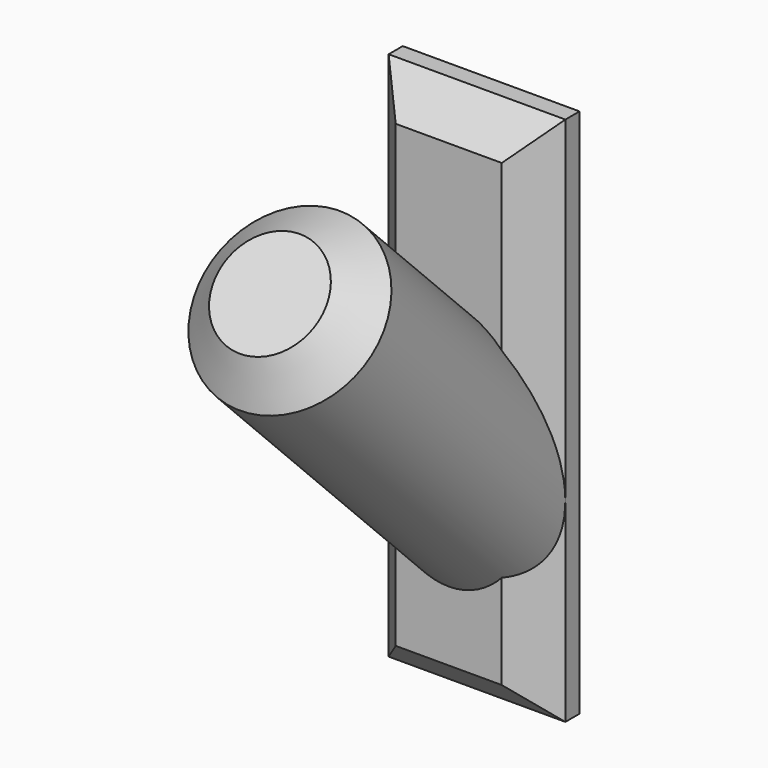
from build123d import *

# Parameters (mm, degrees)
F0_W          = 10
F0_H          = 30
F1_DEPTH      = 3
F4_R          = 5
F5_DEPTH      = 20
F5_DEPTH_BACK = 5
F6_T1_DEPTH   = 20.2867319519
F6_T6_DEPTH   = 22.1433659759
F6_S7_R       = 5
F6_T8_DEPTH   = 13
F6_T14_DEPTH  = 22.1433659759
F6_S15_R      = 5
F6_T16_DEPTH  = 13
F6_T20_DEPTH  = 18.1433659759
F6_S21_R      = 5
F6_T22_DEPTH  = 11
F6_T26_DEPTH  = 18.1433659759
F6_S27_R      = 5
F6_T28_DEPTH  = 11
F7_DEPTH      = 25


# Not quite as in the source:
# - a fillet or chamfer that OpenCascade refuses, or shapes differently, is made with other operations: its cross-section is extruded or revolved along the edge and cut away or added


with BuildPart() as f1:
    # F0 (on Front) → F1 (new body)
    with BuildSketch(Plane.XZ):
        with Locations((0, 5)):
            Rectangle(F0_W, F0_H)
    extrude(amount=F1_DEPTH)

    # F4 (on face) → F5 (join, two sides)
    with BuildSketch(Plane(origin=(0, -1.5, 1.5), x_dir=(1, 0, 0), z_dir=(0, -0.7071067812, 0.7071067812))) as f5_sk:
        Circle(F4_R)
    extrude(amount=F5_DEPTH)
    extrude(f5_sk.sketch, amount=-F5_DEPTH_BACK)

    # F6: chamfer of 2 on 5 edges, made by hand

    # F6_s2 → F6_t1 (cut)
    with BuildSketch(Plane.YZ.offset(-10.1433659759)):
        Polygon((-1, 20), (-3, 18), (-3, 20), align=None)
        Polygon((-3, -8), (-1, -10), (-3, -10), align=None)
    extrude(amount=F6_T1_DEPTH, mode=Mode.SUBTRACT)


with BuildPart() as f6_tool4:
    # F6_s5 → F6_t6 (new body)
    with BuildSketch(Plane.XY.offset(25.1433659759)):
        Polygon((-3, -3), (-5, -1), (-5, -3), align=None)
    extrude(amount=-F6_T6_DEPTH)

    # F6_s7 → F6_t8 (cut, symmetric)
    with BuildSketch(Plane(origin=(0, -8.0610173055, 8.0610173055), x_dir=(1, 0, 0), z_dir=(0, 0.7071067812, -0.7071067812))):
        Circle(F6_S7_R)
    extrude(amount=F6_T8_DEPTH, both=True, mode=Mode.SUBTRACT)


with BuildPart() as f1_1:
    add(f1.part)

    # F6_t3: cut F6_tool4
    add(f6_tool4.part, mode=Mode.SUBTRACT)

    # F6_s9 → F6_t10 (revolve, cut)
    with BuildSketch(Plane(origin=(0, 0, 0), x_dir=(1, 0, 0), z_dir=(0, -0.7071067812, -0.7071067812))):
        Polygon((5, 20.1213203436), (3, 22.1213203436), (5, 22.1213203436), align=None)
    revolve(axis=Axis((0, -15.6421356237, 15.6421356237), (0, -0.7071067812, 0.7071067812)), mode=Mode.SUBTRACT)


with BuildPart() as f6_tool12:
    # F6_s13 → F6_t14 (new body)
    with BuildSketch(Plane.XY.offset(3)):
        Polygon((3, -3), (5, -1), (5, -3), align=None)
    extrude(amount=F6_T14_DEPTH)

    # F6_s15 → F6_t16 (cut, symmetric)
    with BuildSketch(Plane(origin=(0, -8.0610173055, 8.0610173055), x_dir=(1, 0, 0), z_dir=(0, 0.7071067812, -0.7071067812))):
        Circle(F6_S15_R)
    extrude(amount=F6_T16_DEPTH, both=True, mode=Mode.SUBTRACT)


with BuildPart() as f1_2:
    add(f1_1.part)

    # F6_t11: cut F6_tool12
    add(f6_tool12.part, mode=Mode.SUBTRACT)


with BuildPart() as f6_tool18:
    # F6_s19 → F6_t20 (new body)
    with BuildSketch(Plane.XY.offset(-15.1433659759)):
        Polygon((3, -3), (5, -1), (5, -3), align=None)
    extrude(amount=F6_T20_DEPTH)

    # F6_s21 → F6_t22 (cut, symmetric)
    with BuildSketch(Plane(origin=(0, 2.0506096654, -2.0506096654), x_dir=(1, 0, 0), z_dir=(0, 0.7071067812, -0.7071067812))):
        Circle(F6_S21_R)
    extrude(amount=F6_T22_DEPTH, both=True, mode=Mode.SUBTRACT)


with BuildPart() as f1_3:
    add(f1_2.part)

    # F6_t17: cut F6_tool18
    add(f6_tool18.part, mode=Mode.SUBTRACT)


with BuildPart() as f6_tool24:
    # F6_s25 → F6_t26 (new body)
    with BuildSketch(Plane.XY.offset(3)):
        Polygon((-3, -3), (-5, -1), (-5, -3), align=None)
    extrude(amount=-F6_T26_DEPTH)

    # F6_s27 → F6_t28 (cut, symmetric)
    with BuildSketch(Plane(origin=(0, 2.0506096654, -2.0506096654), x_dir=(1, 0, 0), z_dir=(0, 0.7071067812, -0.7071067812))):
        Circle(F6_S27_R)
    extrude(amount=F6_T28_DEPTH, both=True, mode=Mode.SUBTRACT)


with BuildPart() as f1_4:
    add(f1_3.part)

    # F6_t23: cut F6_tool24
    add(f6_tool24.part, mode=Mode.SUBTRACT)

    # F0 (on Front) → F7 (cut)
    with BuildSketch(Plane.XZ):
        with Locations((0, 5)):
            Rectangle(F0_W, F0_H)
    extrude(amount=-F7_DEPTH, mode=Mode.SUBTRACT)


solid = f1_4.part
